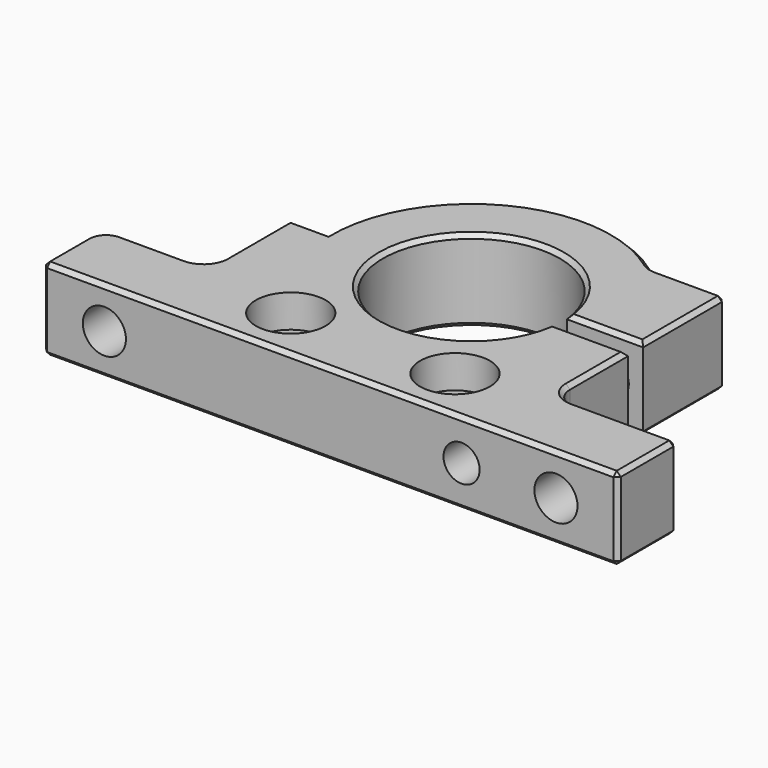
from build123d import *

# Parameters (mm, degrees)
F0_W            = 9.2476086318
F0_H            = 25
F1_DEPTH        = 20
F3_D            = 8.8
F3_DEPTH        = 40.701
F4_D            = 9
F4_DEPTH        = 37.301
F6_D            = 10.5
F7_R            = 5
F8_SIZE         = 1
F10_D           = 8
F10_CBORE_D     = 17
F10_CBORE_DEPTH = 8


# Not quite as in the source:
# - a feature names something its author has since deleted; it is built from what else it names


with BuildPart() as f1:
    # F0 (on Top) → F1 (new body)
    with BuildSketch(Plane.XY):
        with BuildLine():
            ThreePointArc((21.4269106499, -2.3), (-21.55, 0), (21.4269106499, 2.3))
            Line((21.4269106499, 2.3), (40, 2.3))
            Line((40, 2.3), (40, 27.2765494883))
            Line((40, 27.2765494883), (21.9314807528, 27.2765494883))
            ThreePointArc((21.9314807528, 27.2765494883), (-15.122800231, 31.5642347155), (-35, 0))
            ThreePointArc((-35, 0), (-1.1506219411, -34.9810815892), (34.9243468085, -2.3))
            Line((34.9243468085, -2.3), (21.4269106499, -2.3))
        make_face()
        with BuildLine():
            Line((40, -2.3), (34.9243468085, -2.3))
            ThreePointArc((34.9243468085, -2.3), (-1.1506219411, -34.9810815892), (-35, 0))
            Line((-35, 0), (-35, -25))
            Line((-35, -25), (-44.2476086318, -25))
            Line((-44.2476086318, -25), (-70, -25))
            Line((-70, -25), (-70, -43))
            Line((-70, -43), (70, -43))
            Line((70, -43), (70, -25))
            Line((70, -25), (40, -25))
            Line((40, -25), (40, -2.3))
        make_face()
        with Locations((-39.6238043159, -12.5)):
            Rectangle(F0_W, F0_H)
    extrude(amount=F1_DEPTH)

    # F3 (through all, one way)
    with BuildSketch(Plane(origin=(0, -2.3, 0), x_dir=(-1, 0, 0), z_dir=(0, 1, 0))):
        with Locations((-32, 10)):
            Circle(F3_D / 2)
    extrude(amount=-F3_DEPTH, mode=Mode.SUBTRACT)

    # F4 (through all, one way)
    with BuildSketch(Plane(origin=(0, -2.3, 0), x_dir=(-1, 0, 0), z_dir=(0, -1, 0))):
        with Locations((-32, -10)):
            Circle(F4_D / 2)
    extrude(amount=-F4_DEPTH, mode=Mode.SUBTRACT)

    # F6 (through all)
    with Locations(Plane(origin=(0, -25, 0), x_dir=(-1, 0, 0), z_dir=(0, 1, 0))):
        with Locations((55, 10), (-55, 10)):
            Hole(F6_D / 2)

    # F7
    f7_edges = [f1.edges().sort_by_distance(p)[0] for p in [
        (40, -25, 10),
        (21.931481, 27.276549, 10),
        (-44.247609, -25, 10),
        (-70, -25, 10),
    ]]
    fillet(f7_edges, radius=F7_R)

    # F8
    f8_edges = [f1.edges().sort_by_distance(p)[0] for p in [
        (31.813386, 27.276549, 20),
        (22.073202, 27.524032, 20),
        (40, 14.788275, 20),
        (-15.833984, 31.213538, 20),
        (30.713455, 2.3, 20),
        (-39.623804, 0, 20),
        (-21.55, 0, 20),
        (-44.247609, -10, 20),
        (30.713455, -2.3, 20),
        (-45.712075, -23.535534, 20),
        (40, -11.15, 20),
        (-57.123804, -25, 20),
        (41.464466, -23.535534, 20),
        (-68.535534, -26.464466, 20),
        (57.5, -25, 20),
        (-70, -36.5, 20),
        (70, -34, 20),
        (0, -43, 20),
        (31.813386, 27.276549, 0),
        (22.073202, 27.524032, 0),
        (40, 14.788275, 0),
        (-15.833984, 31.213538, 0),
        (30.713455, 2.3, 0),
        (-39.623804, 0, 0),
        (-21.55, 0, 0),
        (-44.247609, -10, 0),
        (30.713455, -2.3, 0),
        (-45.712075, -23.535534, 0),
        (40, -11.15, 0),
        (-57.123804, -25, 0),
        (41.464466, -23.535534, 0),
        (-68.535534, -26.464466, 0),
        (57.5, -25, 0),
        (-70, -36.5, 0),
        (70, -34, 0),
        (0, -43, 0),
        (23.626772, 27.276549, 10),
        (40, 27.276549, 10),
        (36.5, 27.276549, 10),
        (-70, -30, 10),
        (-70, -43, 10),
        (70, -43, 10),
        (70, -25, 10),
    ]]
    chamfer(f8_edges, length=F8_SIZE)

    # F10 (through all)
    with Locations(Plane.XY.offset(20)):
        with Locations((-20, -30), (20, -30)):
            CounterBoreHole(F10_D / 2, F10_CBORE_D / 2, F10_CBORE_DEPTH)


solid = f1.part
